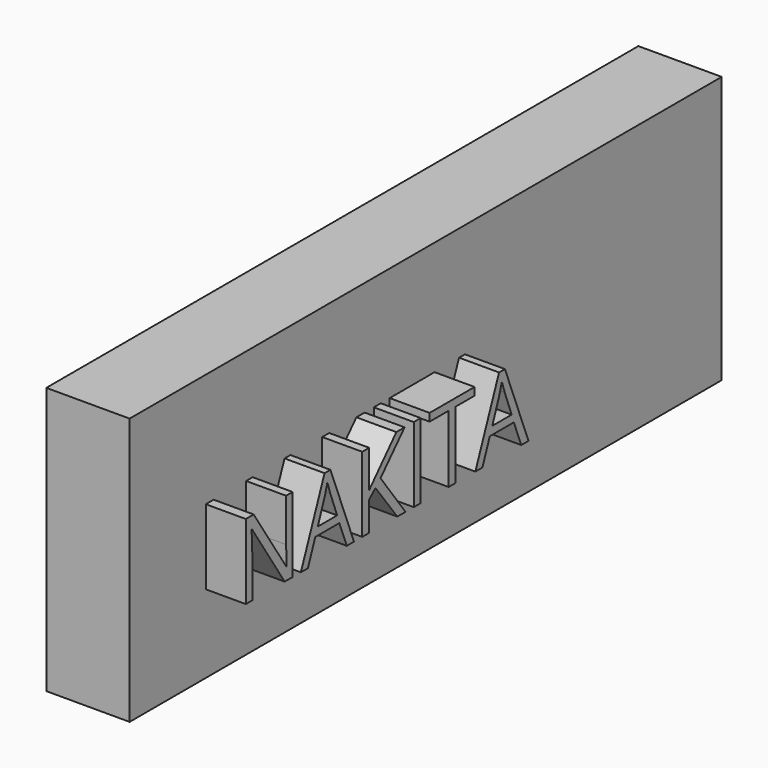
from build123d import *

# Parameters (mm, degrees)
F0_W         = 222.0334410667
F0_H         = 80.1089927554
F1_DEPTH     = 25
F2_TEXT_SIZE = 31.4826268651
F3_DEPTH     = 12


# Not quite as in the source:
# - Text() gives the source's letters only with a copy of the font that has no kerning and outlines rounded to 1/6400 em; it was checked with that copy


with BuildPart() as f1:
    # F0 (on Right) → F1 (new body)
    with BuildSketch(Plane.YZ):
        Rectangle(F0_W, F0_H)
    extrude(amount=F1_DEPTH)

    # F2 (on face) → F3 (join)
    with BuildSketch(Plane.YZ.offset(25)):
        with Locations((-85.5367183685, -16.6453309357)):
            Text('NAKITA', F2_TEXT_SIZE, font='Open Sans', text_align=(TextAlign.LEFT, TextAlign.BOTTOM))
    extrude(amount=F3_DEPTH)


solid = f1.part
